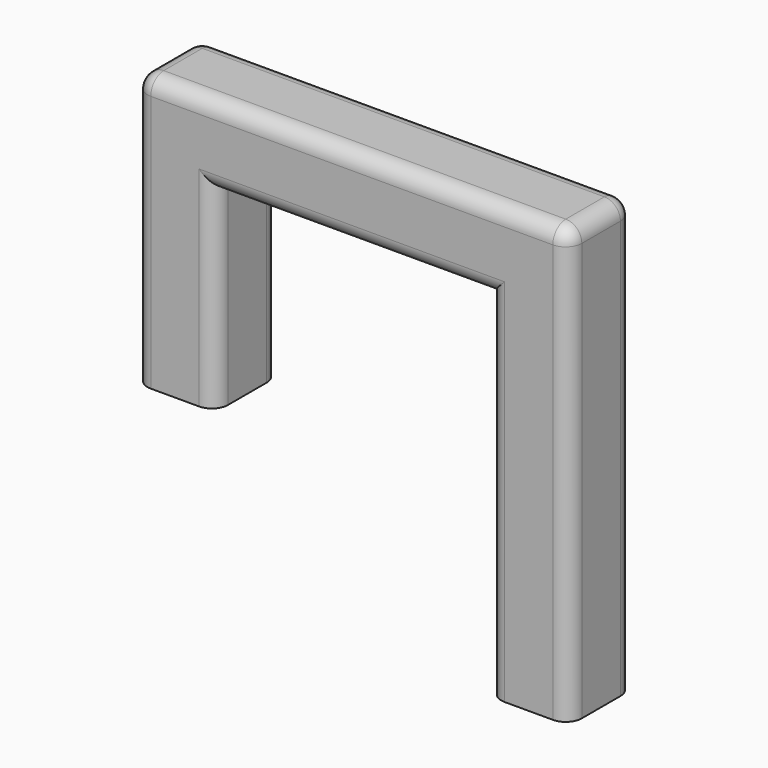
from build123d import *

# Parameters (mm, degrees)
F0_W     = 25
F0_H     = 25
F1_DEPTH = 60
F2_W     = 25
F2_H     = 25
F3_DEPTH = 60
F4_DEPTH = 25
F5_DEPTH = 50
F6_W     = 25
F6_H     = 25
F7_DEPTH = 110
F8_R     = 5


with BuildPart() as f1:
    # F0 (on Top) → F1 (new body)
    with BuildSketch(Plane.XY):
        with Locations((12.5, 12.5)):
            Rectangle(F0_W, F0_H)
    extrude(amount=F1_DEPTH)

    # F2 (on face) → F3 (join)
    with BuildSketch(Plane.YZ.offset(25)):
        with Locations((12.5, 47.5)):
            Rectangle(F2_W, F2_H)
    extrude(amount=F3_DEPTH)

    # F4 (add): a face of the model
    f4_faces = [f1.faces().sort_by_distance(p)[0] for p in [
        (12.5, 12.5, 0),
    ]]
    extrude(f4_faces, amount=F4_DEPTH)

    # F5 (add): a face of the model
    f5_faces = [f1.faces().sort_by_distance(p)[0] for p in [
        (85, 12.5, 47.5),
    ]]
    extrude(f5_faces, amount=F5_DEPTH)

    # F6 (on face) → F7 (join)
    with BuildSketch(Plane(origin=(0, 0, 35), x_dir=(1, 0, 0), z_dir=(0, 0, -1))):
        with Locations((122.5, -12.5)):
            Rectangle(F6_W, F6_H)
    extrude(amount=F7_DEPTH)

    # F8
    f8_edges = [f1.edges().sort_by_distance(p)[0] for p in [
        (67.5, 0, 60),
        (67.5, 25, 60),
        (25, 0, 5),
        (25, 25, 5),
        (0, 0, 17.5),
        (0, 25, 17.5),
        (67.5, 0, 35),
        (135, 0, -7.5),
        (135, 25, -7.5),
        (135, 12.5, 60),
        (0, 12.5, 60),
        (67.5, 25, 35),
        (110, 0, -20),
    ]]
    fillet(f8_edges, radius=F8_R)


solid = f1.part
